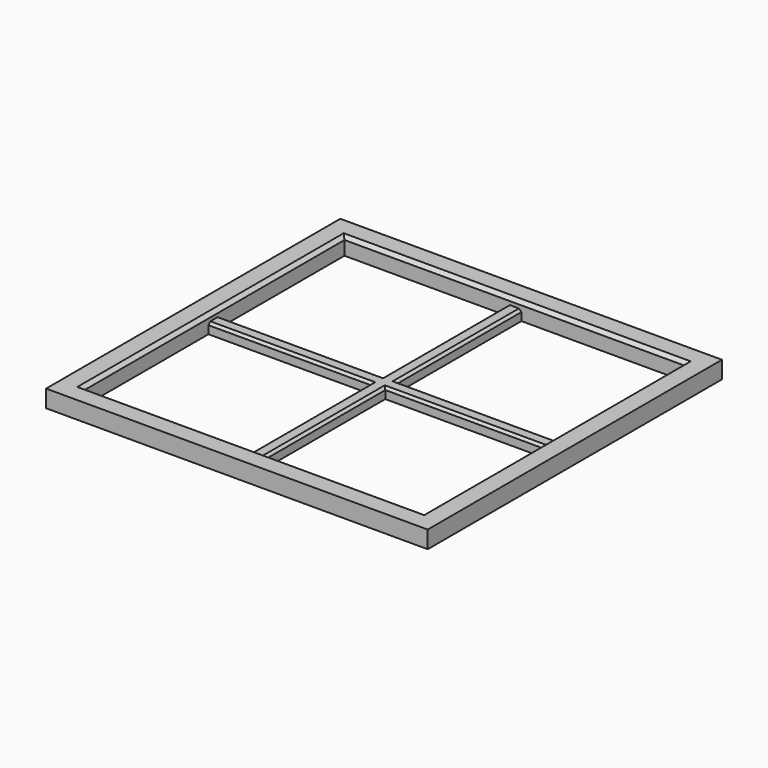
from build123d import *

# Parameters (mm, degrees)
F0_W     = 1100
F0_H     = 1060
F1_DEPTH = 50
F2_SIZE  = 10
F3_DEPTH = 30
F4_SIZE  = 7


# Not quite as in the source:
# - a feature names something its author has since deleted; it is built from what else it names


with BuildPart() as f1:
    # F0 (on Top) → F1 (new body)
    with BuildSketch(Plane.XY):
        with Locations((172.132343931, -6.6134499709)):
            Rectangle(F0_W, F0_H)
        Polygon((-317.867656069, 13.3865500291), (-317.867656069, 463.3865500291), (152.132343931, 463.3865500291), (192.132343931, 463.3865500291), (662.132343931, 463.3865500291), (662.132343931, 15.2047318473), (662.132343931, -24.7952681527), (662.132343931, -476.6134499709), (190.3141621128, -476.6134499709), (150.3141621128, -476.6134499709), (-317.867656069, -476.6134499709), (-317.867656069, -26.6134499709), align=None, mode=Mode.SUBTRACT)
    extrude(amount=F1_DEPTH)

    # F2
    f2_edges = [f1.edges().sort_by_distance(p)[0] for p in [
        (-317.867656, -6.61345, 50),
        (172.132344, 463.38655, 50),
        (662.132344, -6.61345, 50),
        (172.132344, -476.61345, 50),
    ]]
    chamfer(f2_edges, length=F2_SIZE)


with BuildPart() as f3:
    # F0 (on Top) → F3 (new body)
    with BuildSketch(Plane.XY):
        Polygon((192.132343931, 463.3865500291), (152.132343931, 463.3865500291), (152.132343931, 13.3865500291), (-317.867656069, 13.3865500291), (-317.867656069, -26.6134499709), (150.3141621128, -26.6134499709), (150.3141621128, -476.6134499709), (190.3141621128, -476.6134499709), (190.3141621128, -24.7952681527), (662.132343931, -24.7952681527), (662.132343931, 15.2047318473), (192.132343931, 15.2047318473), align=None)
    extrude(amount=F3_DEPTH)

    # F4
    f4_edges = [f3.edges().sort_by_distance(p)[0] for p in [
        (-83.776747, -26.61345, 30),
        (-82.867656, 13.38655, 30),
        (152.132344, 238.38655, 30),
        (192.132344, 239.295641, 30),
        (426.223253, -24.795268, 30),
        (427.132344, 15.204732, 30),
        (190.314162, -250.704359, 30),
        (150.314162, -251.61345, 30),
    ]]
    chamfer(f4_edges, length=F4_SIZE)


solid = Compound([f1.part, f3.part])
